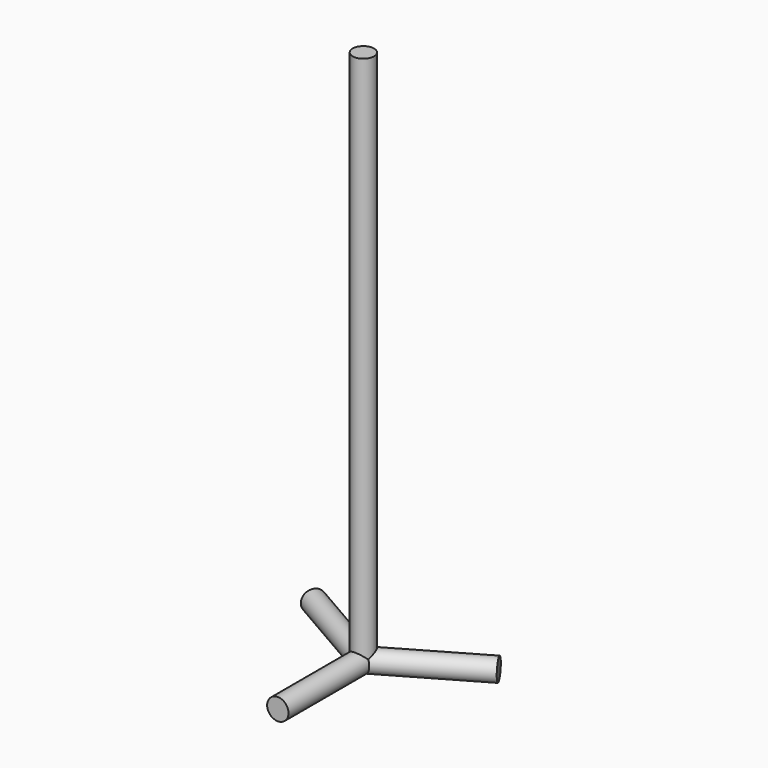
from build123d import *

# Parameters (mm, degrees)
F0_R     = 2.5
F1_DEPTH = 25
F3_COUNT = 3
F2_R     = 2.5
F4_DEPTH = 125


with BuildPart() as f1:
    # F0 (on Front) → F1 (new body)
    with BuildSketch(Plane.XZ):
        Circle(F0_R)
    extrude(amount=F1_DEPTH)


with BuildPart() as f3_1:
    # F3: instance of F1
    add(f1.part.rotate(Axis((0, 0, 0), (0, 0, 1)), 1 * 360 / F3_COUNT))


with BuildPart() as f3_2:
    # F3: instance of F1
    add(f1.part.rotate(Axis((0, 0, 0), (0, 0, 1)), 2 * 360 / F3_COUNT))


with BuildPart() as f1_1:
    add(f1.part)

    add(f3_1.part)  # F4 merges F3_1

    add(f3_2.part)  # F4 merges F3_2
    # F2 (on Top) → F4 (join)
    with BuildSketch(Plane.XY):
        Circle(F2_R)
    extrude(amount=F4_DEPTH)


solid = f1_1.part
